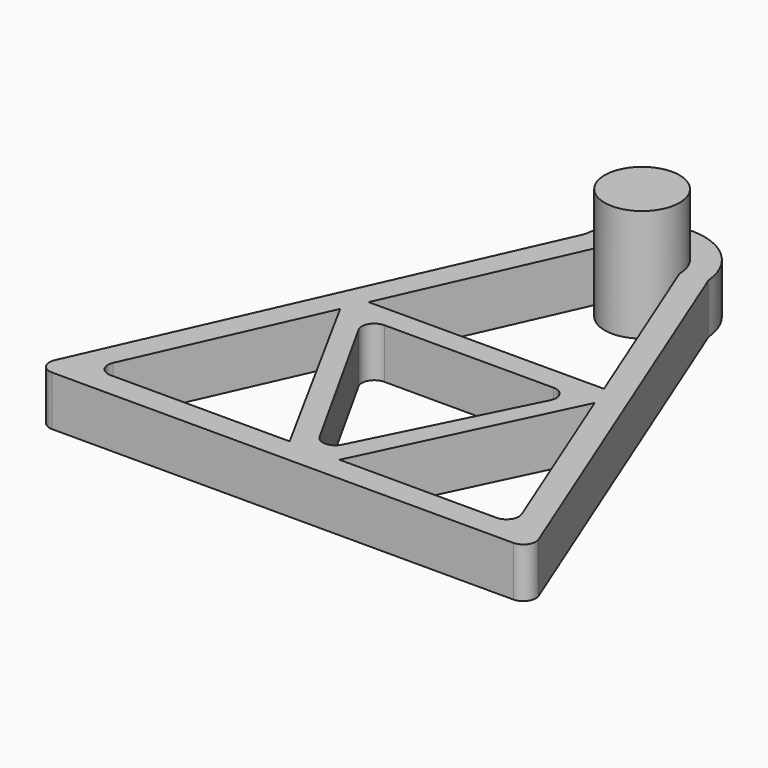
from build123d import *

# Parameters (mm, degrees)
F1_DEPTH = 20
F2_R     = 15
F3_DEPTH = 25


with BuildPart() as f1:
    # F0 (on Top) → F1 (new body)
    with BuildSketch(Plane.XY):
        with BuildLine():
            Line((66.0472436046, -26.2565443359), (-2.0937833608, 144.0460289628))
            ThreePointArc((-2.0937833608, 144.0460289628), (-26.8847617752, 166.8857654042), (-51.8857822677, 144.2761403347))
            Line((-51.8857822677, 144.2761403347), (-128.0604405721, -26.0728991835))
            ThreePointArc((-128.0604405721, -26.0728991835), (-127.6915622894, -30.833770725), (-123.4960085584, -33.1139676273))
            Line((-123.4960085584, -33.1139676273), (61.4050481416, -33.1139676273))
            ThreePointArc((61.4050481416, -33.1139676273), (65.5455261609, -30.9169021202), (66.0472436046, -26.2565443359))
        make_face()
        with BuildLine():
            Line((-36.2713433227, -23.1139676273), (-108.0700619725, -23.1139676273))
            ThreePointArc((-108.0700619725, -23.1139676273), (-112.2656157035, -20.833770725), (-112.6344939862, -16.0728991835))
            Line((-112.6344939862, -16.0728991835), (-80.009586342, 56.8860323727))
            Line((-80.009586342, 56.8860323727), (-75.9274494544, 66.0148964001))
            Line((-75.9274494544, 66.0148964001), (-42.0002968609, 141.8860323727))
            ThreePointArc((-42.0002968609, 141.8860323727), (-37.6068985787, 152.4926340905), (-27.0002968609, 156.8860323727))
            ThreePointArc((-27.0002968609, 156.8860323727), (-16.3936951431, 152.4926340905), (-12.0002968609, 141.8860323727))
            Line((-12.0002968609, 141.8860323727), (18.2948376146, 66.1704232987))
            Line((18.2948376146, 66.1704232987), (22.0096841973, 56.8860323727))
            Line((22.0096841973, 56.8860323727), (51.2753035904, -16.2565443359))
            ThreePointArc((51.2753035904, -16.2565443359), (50.7735861467, -20.9169021202), (46.6331081274, -23.1139676273))
            Line((46.6331081274, -23.1139676273), (-16.2713433227, -23.1139676273))
            Line((-16.2713433227, -23.1139676273), (-36.2713433227, -23.1139676273))
        make_face(mode=Mode.SUBTRACT)
        Polygon((-80.009586342, 56.8860323727), (-36.2713433227, -23.1139676273), (-16.2713433227, -23.1139676273), (22.0096841973, 56.8860323727), (18.2948376146, 66.1704232987), (-75.9274494544, 66.0148964001), align=None)
        with BuildLine():
            Line((-62.3322616112, 56.8860323727), (5.5765360215, 56.8860323727))
            ThreePointArc((5.5765360215, 56.8860323727), (9.8288943227, 54.5161367201), (10.0501944434, 49.6530119241))
            Line((10.0501944434, 49.6530119241), (-22.0404632685, -14.6377746762))
            ThreePointArc((-22.0404632685, -14.6377746762), (-26.4008005729, -17.403469895), (-30.8819908215, -14.8382125186))
            Line((-30.8819908215, -14.8382125186), (-66.7001307422, 49.4525740817))
            ThreePointArc((-66.7001307422, 49.4525740817), (-66.6431368968, 54.4190847355), (-62.3322616112, 56.8860323727))
        make_face(mode=Mode.SUBTRACT)
        with BuildLine():
            ThreePointArc((-27.0002968609, 156.8860323727), (-37.6068985787, 152.4926340905), (-42.0002968609, 141.8860323727))
            ThreePointArc((-42.0002968609, 141.8860323727), (-27.0002968609, 126.8860323727), (-12.0002968609, 141.8860323727))
            ThreePointArc((-12.0002968609, 141.8860323727), (-16.3936951431, 152.4926340905), (-27.0002968609, 156.8860323727))
        make_face()
    extrude(amount=F1_DEPTH)

    # F2 (on face) → F3 (join)
    with BuildSketch(Plane.XY.offset(20)):
        with Locations((-27.0002968609, 141.8860323727)):
            Circle(F2_R)
    extrude(amount=F3_DEPTH)


solid = f1.part
